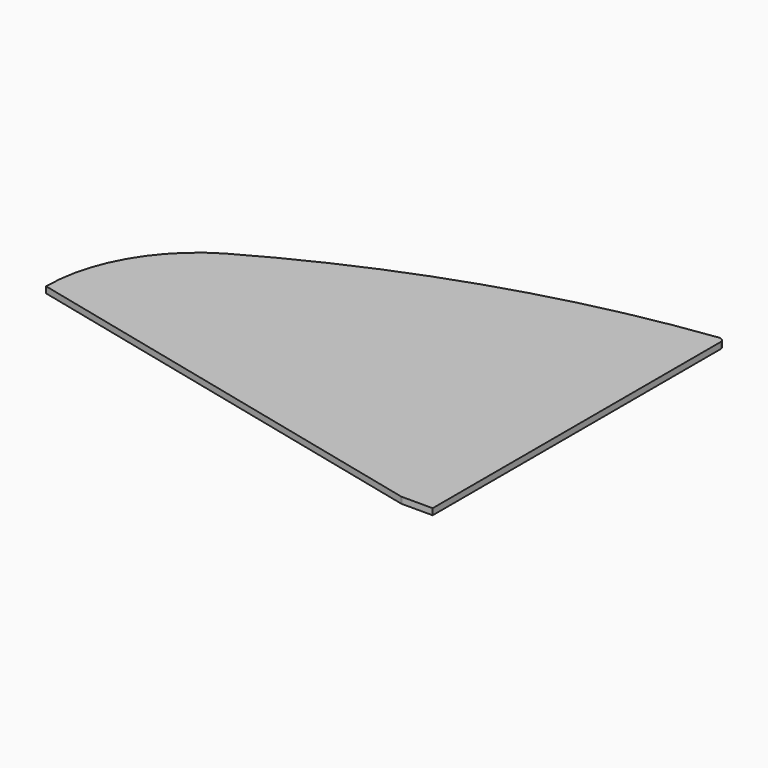
from build123d import *

# Parameters (mm, degrees)
F1_DEPTH = 6
F2_R     = 5


with BuildPart() as f1:
    # F0 (on Top) → F1 (new body)
    with BuildSketch(Plane.XY):
        with BuildLine():
            Line((195, -175), (225, -175))
            Line((225, -175), (225, 175))
            ThreePointArc((225, 175), (29.4969127553, 131.3574891295), (-153.5716205835, 50.0430501997))
            ThreePointArc((-153.5716205835, 50.0430501997), (-205.8843017039, -2.9969136264), (-225, -75))
            Line((-225, -75), (195, -175))
        make_face()
    extrude(amount=F1_DEPTH)

    # F2
    f2_edges = [f1.edges().sort_by_distance(p)[0] for p in [
        (225, 175, 3),
        (195, -175, 3),
    ]]
    fillet(f2_edges, radius=F2_R)


solid = f1.part
